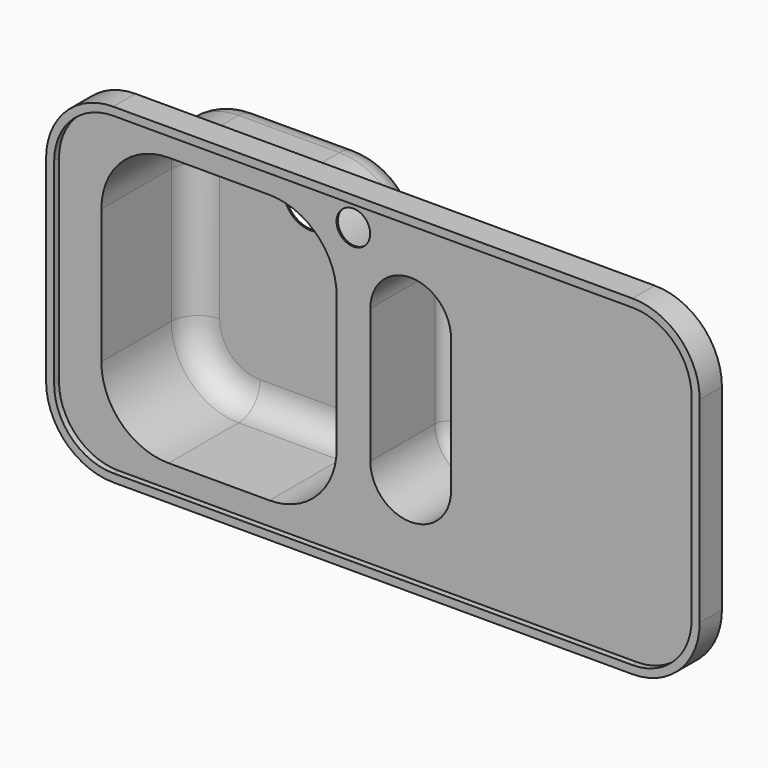
from build123d import *

# Parameters (mm, degrees)
F1_DEPTH     = 300
F2_W         = 350
F2_H         = 400
F3_DEPTH     = 170
F4_R         = 40
F5_T1_DEPTH  = 170
F5_T4_ANGLE  = 90
F5_T6_ANGLE  = 90
F5_T8_ANGLE  = 90
F5_T10_ANGLE = 90
F7_DEPTH     = 140
F8_R         = 20
F10_DEPTH    = 9
F11_T        = -2.5
F12_DEPTH    = 267.6571849734
F13_R        = 40
F14_DEPTH    = 2.501
F15_R        = 25
F16_DEPTH    = 32.501
F17_R        = 25
F18_DEPTH    = 172.501


# Not quite as in the source:
# - a fillet or chamfer that OpenCascade refuses, or shapes differently, is made with other operations: its cross-section is extruded or revolved along the edge and cut away or added


with BuildPart() as f1:
    # F0 (on Front) → F1 (new body)
    with BuildSketch(Plane.XZ):
        with BuildLine():
            Line((-386, -246), (386, -246))
            ThreePointArc((386, -246), (456.7106781187, -216.7106781187), (486, -146))
            Line((486, -146), (486, 146))
            ThreePointArc((486, 146), (456.7106781187, 216.7106781187), (386, 246))
            Line((386, 246), (-386, 246))
            ThreePointArc((-386, 246), (-456.7106781187, 216.7106781187), (-486, 146))
            Line((-486, 146), (-486, -146))
            ThreePointArc((-486, -146), (-456.7106781187, -216.7106781187), (-386, -246))
        make_face()
    extrude(amount=-F1_DEPTH)

    # F2 (on face) → F3 (cut)
    with BuildSketch(Plane.XZ):
        with Locations((-236, 0)):
            Rectangle(F2_W, F2_H)
    extrude(amount=-F3_DEPTH, mode=Mode.SUBTRACT)

    # F4
    f4_edges = [f1.edges().sort_by_distance(p)[0] for p in [
        (-61, 170, 0),
        (-236, 170, 200),
        (-411, 170, 0),
        (-236, 170, -200),
    ]]
    fillet(f4_edges, radius=F4_R)

    # F5: fillet of radius 100 on 4 edges, made by hand

    # F5_s2 → F5_t1 (join)
    with BuildSketch(Plane.XZ.offset(-170)):
        with BuildLine():
            ThreePointArc((-311, 200), (-381.7106781187, 170.7106781187), (-411, 100))
            Line((-411, 100), (-411, 200))
            Line((-411, 200), (-311, 200))
        make_face()
        with BuildLine():
            ThreePointArc((-311, -200), (-381.7106781187, -170.7106781187), (-411, -100))
            Line((-411, -100), (-411, -200))
            Line((-411, -200), (-311, -200))
        make_face()
        with BuildLine():
            ThreePointArc((-61, 100), (-90.2893218813, 170.7106781187), (-161, 200))
            Line((-161, 200), (-61, 200))
            Line((-61, 200), (-61, 100))
        make_face()
        with BuildLine():
            ThreePointArc((-61, -100), (-90.2893218813, -170.7106781187), (-161, -200))
            Line((-161, -200), (-61, -200))
            Line((-61, -200), (-61, -100))
        make_face()
    extrude(amount=F5_T1_DEPTH)

    # F5_s3 → F5_t4 (revolve)
    with BuildSketch(Plane.XY.offset(-100)):
        with BuildLine():
            ThreePointArc((-101, 170), (-72.7157287525, 158.2842712475), (-61, 130))
            Line((-61, 130), (-61, 170))
            Line((-61, 170), (-101, 170))
        make_face()
    revolve(axis=Axis((-161, 170, -100), (0, 1, 0)), revolution_arc=F5_T4_ANGLE)

    # F5_s5 → F5_t6 (revolve)
    with BuildSketch(Plane.YZ.offset(-161)):
        with BuildLine():
            ThreePointArc((170, 160), (158.2842712475, 188.2842712475), (130, 200))
            Line((130, 200), (170, 200))
            Line((170, 200), (170, 160))
        make_face()
    revolve(axis=Axis((-161, 170, 100), (0, 1, 0)), revolution_arc=F5_T6_ANGLE)

    # F5_s7 → F5_t8 (revolve)
    with BuildSketch(Plane.YZ.offset(-311)):
        with BuildLine():
            ThreePointArc((170, -160), (158.2842712475, -188.2842712475), (130, -200))
            Line((130, -200), (170, -200))
            Line((170, -200), (170, -160))
        make_face()
    revolve(axis=Axis((-311, 170, -100), (0, 1, 0)), revolution_arc=F5_T8_ANGLE)

    # F5_s9 → F5_t10 (revolve)
    with BuildSketch(Plane.XY.offset(100)):
        with BuildLine():
            ThreePointArc((-371, 170), (-399.2842712475, 158.2842712475), (-411, 130))
            Line((-411, 130), (-411, 170))
            Line((-411, 170), (-371, 170))
        make_face()
    revolve(axis=Axis((-311, 170, 100), (0, 1, 0)), revolution_arc=F5_T10_ANGLE)

    # F6 (on face) → F7 (cut)
    with BuildSketch(Plane.XZ):
        with BuildLine():
            ThreePointArc((-11, -100), (49, -160), (109, -100))
            Line((109, -100), (109, 100))
            ThreePointArc((109, 100), (49, 160), (-11, 100))
            Line((-11, 100), (-11, -100))
        make_face()
    extrude(amount=-F7_DEPTH, mode=Mode.SUBTRACT)

    # F8
    f8_edges = [f1.edges().sort_by_distance(p)[0] for p in [
        (49, 140, -160),
        (109, 140, 0),
        (49, 140, 160),
        (-11, 140, 0),
    ]]
    fillet(f8_edges, radius=F8_R)

    # F9 (on face) → F10 (join)
    with BuildSketch(Plane.XZ):
        with BuildLine():
            Line((386, 246), (-386, 246))
            ThreePointArc((-386, 246), (-456.7106781187, 216.7106781187), (-486, 146))
            Line((-486, 146), (-486, -146))
            ThreePointArc((-486, -146), (-456.7106781187, -216.7106781187), (-386, -246))
            Line((-386, -246), (386, -246))
            ThreePointArc((386, -246), (456.7106781187, -216.7106781187), (486, -146))
            Line((486, -146), (486, 146))
            ThreePointArc((486, 146), (456.7106781187, 216.7106781187), (386, 246))
        make_face()
        with BuildLine():
            ThreePointArc((386, 234), (448.2253967444, 208.2253967444), (474, 146))
            Line((474, 146), (474, -146))
            ThreePointArc((474, -146), (448.2253967444, -208.2253967444), (386, -234))
            Line((386, -234), (-386, -234))
            ThreePointArc((-386, -234), (-448.2253967444, -208.2253967444), (-474, -146))
            Line((-474, -146), (-474, 146))
            ThreePointArc((-474, 146), (-448.2253967444, 208.2253967444), (-386, 234))
            Line((-386, 234), (386, 234))
        make_face(mode=Mode.SUBTRACT)
    extrude(amount=F10_DEPTH)

    # F11
    f11_openings = [f1.faces().sort_by_distance(p)[0] for p in [
        (0, 300, 0),
    ]]
    offset(amount=F11_T, openings=f11_openings, kind=Kind.INTERSECTION)

    # F12 (cut): a face of the model
    f12_faces = [f1.faces().sort_by_distance(p)[0] for p in [
        (0, 300, -244.9105744633),
    ]]
    extrude(f12_faces, amount=-F12_DEPTH, mode=Mode.SUBTRACT)

    # F13 (on face) → F14 (cut, through all)
    with BuildSketch(Plane.XZ.offset(-170)):
        with Locations((-236, 100)):
            Circle(F13_R)
    extrude(amount=-F14_DEPTH, mode=Mode.SUBTRACT)

    # F15 (on face) → F16 (cut, through all)
    with BuildSketch(Plane.XZ.offset(-140)):
        with Locations((49, 100)):
            Circle(F15_R)
    extrude(amount=-F16_DEPTH, mode=Mode.SUBTRACT)

    # F17 (on face) → F18 (cut, through all)
    with BuildSketch(Plane.XZ):
        with Locations((-36.2374484539, 197.7449208498)):
            Circle(F17_R)
    extrude(amount=-F18_DEPTH, mode=Mode.SUBTRACT)


solid = f1.part
